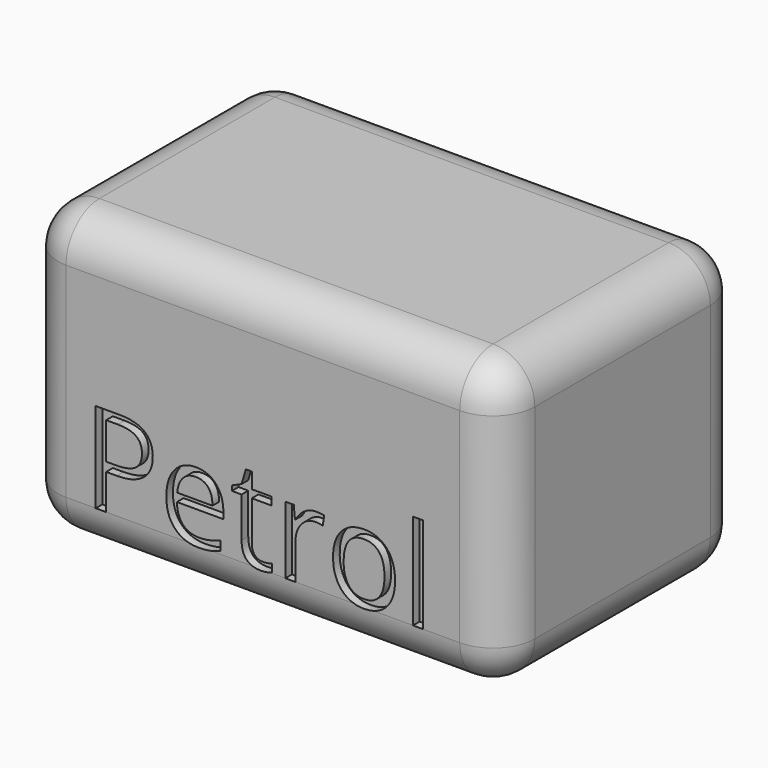
from build123d import *

# Parameters (mm, degrees)
F0_W         = 572
F0_H         = 345
F1_DEPTH     = 363
F2_R         = 50
F3_TEXT_SIZE = 151.1734152834
F4_DEPTH     = 10


# Not quite as in the source:
# - Text() gives the source's letters only with a copy of the font that has no kerning and outlines rounded to 1/6400 em; it was checked with that copy


with BuildPart() as f1:
    # F0 (on Front) → F1 (new body)
    with BuildSketch(Plane.XZ):
        Rectangle(F0_W, F0_H)
    extrude(amount=F1_DEPTH)

    # F2
    f2_edges = [f1.edges().sort_by_distance(p)[0] for p in [
        (0, -363, -172.5),
        (286, -363, 0),
        (0, -363, 172.5),
        (-286, -363, 0),
        (286, -181.5, -172.5),
        (286, -181.5, 172.5),
        (-286, -181.5, 172.5),
        (0, 0, 172.5),
        (-286, -181.5, -172.5),
        (0, 0, -172.5),
        (286, 0, 0),
        (-286, 0, 0),
    ]]
    fillet(f2_edges, radius=F2_R)

    # F3 (on face) → F4 (cut)
    with BuildSketch(Plane.XZ.offset(363)):
        with Locations((-215.2927858803, -122.5)):
            Text('Petrol', F3_TEXT_SIZE, font='Open Sans', text_align=(TextAlign.LEFT, TextAlign.BOTTOM))
    extrude(amount=-F4_DEPTH, mode=Mode.SUBTRACT)


solid = f1.part
